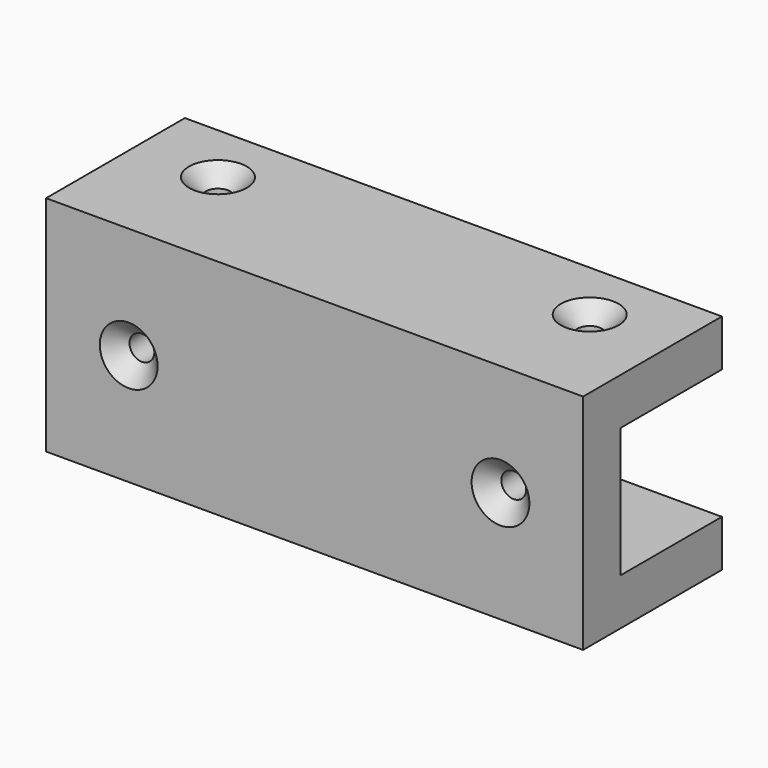
from build123d import *

# Parameters (mm, degrees)
F1_DEPTH      = 65
F2_R          = 1.5
F3_DEPTH      = 21.001
F4_R          = 1.5
F5_DEPTH      = 21.001
F5_DEPTH_BACK = 6.001
F6_SIZE       = 2
F7_W          = 15.7
F7_H          = 15.7
F8_DEPTH      = 65.001


with BuildPart() as f1:
    # F0 (on Right) → F1 (new body)
    with BuildSketch(Plane.YZ):
        Polygon((-7.5, 7.5), (7.5, 7.5), (7.5, 13.5), (-13.5, 13.5), (-13.5, -13.5), (7.5, -13.5), (7.5, -7.5), (-7.5, -7.5), align=None)
    extrude(amount=F1_DEPTH)

    # F2 (on face) → F3 (cut, through all)
    with BuildSketch(Plane.XZ.offset(13.5)):
        with Locations((10, 0)):
            Circle(F2_R)
        with Locations((55, 0)):
            Circle(F2_R)
    extrude(amount=-F3_DEPTH, mode=Mode.SUBTRACT)

    # F4 (on face) → F5 (cut, two sides)
    with BuildSketch(Plane(origin=(0, 0, 7.5), x_dir=(1, 0, 0), z_dir=(0, 0, -1))) as f5_sk:
        with Locations((55, 0)):
            Circle(F4_R)
        with Locations((10, 0)):
            Circle(F4_R)
    extrude(amount=F5_DEPTH, mode=Mode.SUBTRACT)
    extrude(f5_sk.sketch, amount=-F5_DEPTH_BACK, mode=Mode.SUBTRACT)

    # F6
    f6_edges = [f1.edges().sort_by_distance(p)[0] for p in [
        (53.5, 0, 13.5),
        (8.5, 0, 13.5),
        (8.5, -13.5, 0),
        (53.5, -13.5, 0),
        (53.5, 0, -13.5),
        (8.5, 0, -13.5),
    ]]
    chamfer(f6_edges, length=F6_SIZE)

    # F7 (on face) → F8 (cut, through all)
    with BuildSketch(Plane(origin=(0, 0, 0), x_dir=(0, -1, 0), z_dir=(-1, 0, 0))):
        Rectangle(F7_W, F7_H)
    extrude(amount=-F8_DEPTH, mode=Mode.SUBTRACT)


solid = f1.part
